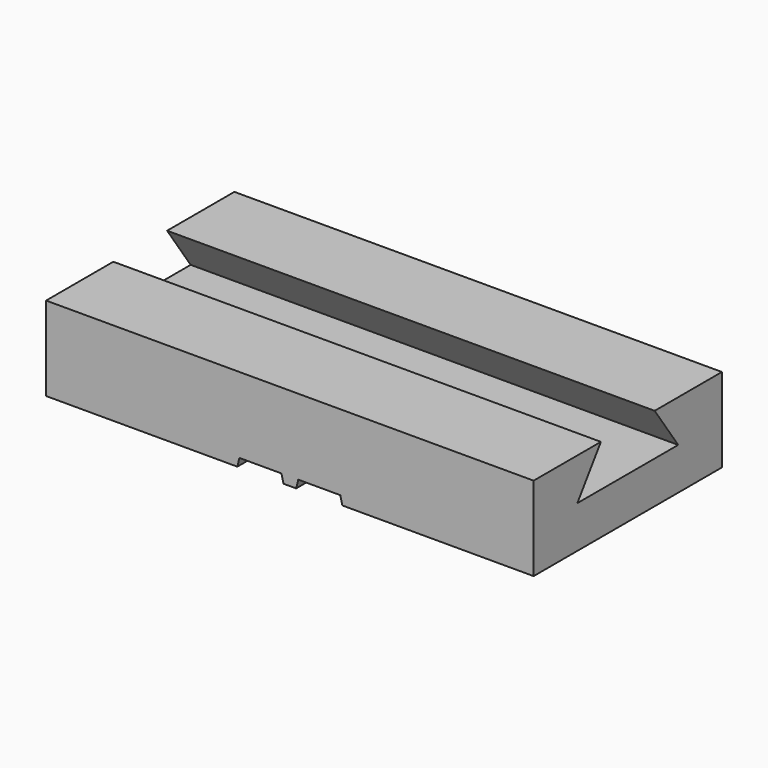
from build123d import *

# Parameters (mm, degrees)
F1_DEPTH = 56
F3_DEPTH = 116
F5_D     = 12
F5_DEPTH = 5
F5_TIP   = 3.6051637142


# Not quite as in the source:
# - a feature names something its author has since deleted; it is built from what else it names


with BuildPart() as f1:
    # F0 (on Front) → F1 (new body)
    with BuildSketch(Plane.XZ):
        Polygon((1.5, 0), (2, 2), (12, 2), (12.5, 0), (58, 0), (58, 20), (-58, 20), (-58, 0), (-12.5, 0), (-12, 2), (-2, 2), (-1.5, 0), (0, 0), align=None)
    extrude(amount=F1_DEPTH)

    # F2 (on face) → F3 (cut, through all)
    with BuildSketch(Plane(origin=(-58, 0, 0), x_dir=(0, -1, 0), z_dir=(-1, 0, 0))):
        Polygon((28, 20), (20.0020753821, 20), (13, 10), (28, 10), align=None)
        Polygon((35.9979246179, 20), (28, 20), (28, 10), (43, 10), align=None)
    extrude(amount=-F3_DEPTH, mode=Mode.SUBTRACT)

    # F5
    with Locations(Plane.XY.offset(10)):
        with Locations((-1.5, -28)):
            Hole(F5_D / 2, depth=F5_DEPTH)
            with Locations((0, 0, -(F5_DEPTH + F5_TIP / 2))):  # 118° drill point
                Cone(0, F5_D / 2, F5_TIP, mode=Mode.SUBTRACT)


solid = f1.part
